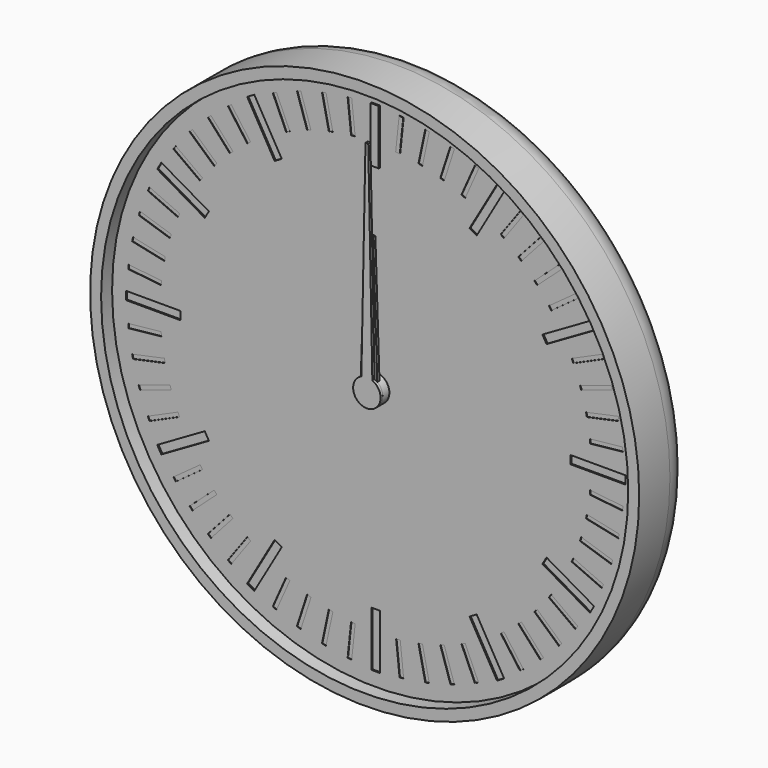
from build123d import *

# Parameters (mm, degrees)
F0_R      = 100
F1_DEPTH  = 24
F2_R      = 10
F3_T      = -4
F4_R      = 5
F4_R_2    = 3
F5_DEPTH  = 2
F6_DEPTH  = 19
F7_DEPTH  = 8
F9_DEPTH  = 4
F11_DEPTH = 4
F12_R     = 5
F12_R_2   = 3
F13_DEPTH = 2
F14_R     = 3
F15_DEPTH = 4
F17_DEPTH = 4
F18_R     = 3
F19_DEPTH = 2
F20_R     = 98
F20_R_2   = 5
F21_DEPTH = 1
F23_R     = 5
F23_R_2   = 3
F24_DEPTH = 2
F25_W     = 3
F25_H     = 20
F25_W_2   = 20
F25_H_2   = 3
F26_DEPTH = 0.5
F27_W     = 1.5
F27_H     = 12
F27_W_2   = 12
F27_H_2   = 1.5
F28_DEPTH = 0.2
F29_DEPTH = 1
F30_DEPTH = 0.4
F31_R     = 5
F31_R_2   = 3
F32_DEPTH = 5
F33_R     = 3
F34_DEPTH = 1
F36_DEPTH = 1


with BuildPart() as f1:
    # F0 (on Front) → F1 (new body)
    with BuildSketch(Plane.XZ):
        Circle(F0_R)
    extrude(amount=F1_DEPTH)

    # F2
    f2_edges = [f1.edges().sort_by_distance(p)[0] for p in [
        (-100, 0, 0),
    ]]
    fillet(f2_edges, radius=F2_R)

    # F3
    f3_openings = [f1.faces().sort_by_distance(p)[0] for p in [
        (0, -24, 0),
    ]]
    offset(amount=F3_T, openings=f3_openings)

    # F4 (on face) → F5 (join)
    with BuildSketch(Plane.XZ.offset(4)):
        Circle(F4_R)
        Circle(F4_R_2, mode=Mode.SUBTRACT)
        with Locations((40, 0)):
            Circle(F4_R)
        with Locations((40, 0)):
            Circle(F4_R_2, mode=Mode.SUBTRACT)
    extrude(amount=F5_DEPTH)


with BuildPart() as f6:
    # F6 (new): a face of the model
    f6_faces = [f1.part.faces().sort_by_distance(p)[0] for p in [
        (0, -4, 0),
    ]]
    extrude(f6_faces, amount=F6_DEPTH)

    # F8 (on face) → F9 (join)
    with BuildSketch(Plane.XZ.offset(6)):
        with BuildLine():
            ThreePointArc((9.2729637667, -1.3794085621), (9.3494561423, -0.6915886375), (9.375, 0))
            ThreePointArc((9.375, 0), (9.3494561423, 0.6915886375), (9.2729637667, 1.3794085621))
            ThreePointArc((9.2729637667, 1.3794085621), (8.9161548403, 2.8970343223), (8.3127812852, 4.3345463782))
            ThreePointArc((8.3127812852, 4.3345463782), (7.5845343223, 5.5104867402), (6.6911892658, 6.566476316))
            ThreePointArc((6.6911892658, 6.566476316), (5.5104867402, 7.5845343223), (4.1773988938, 8.3928519278))
            ThreePointArc((4.1773988938, 8.3928519278), (2.8970343223, 8.9161548403), (1.5536078905, 9.2453733036))
            ThreePointArc((1.5536078905, 9.2453733036), (0, 9.375), (-1.5536078905, 9.2453733036))
            ThreePointArc((-1.5536078905, 9.2453733036), (-2.8970343223, 8.9161548403), (-4.1773988938, 8.3928519278))
            ThreePointArc((-4.1773988938, 8.3928519278), (-5.5104867402, 7.5845343223), (-6.6911892658, 6.566476316))
            ThreePointArc((-6.6911892658, 6.566476316), (-7.5845343223, 5.5104867402), (-8.3127812852, 4.3345463782))
            ThreePointArc((-8.3127812852, 4.3345463782), (-8.9161548403, 2.8970343223), (-9.2729637667, 1.3794085621))
            ThreePointArc((-9.2729637667, 1.3794085621), (-9.375, 0), (-9.2729637667, -1.3794085621))
            ThreePointArc((-9.2729637667, -1.3794085621), (-8.9161548403, -2.8970343223), (-8.3127812852, -4.3345463782))
            ThreePointArc((-8.3127812852, -4.3345463782), (-7.5845343223, -5.5104867402), (-6.6911892658, -6.566476316))
            ThreePointArc((-6.6911892658, -6.566476316), (-5.5104867402, -7.5845343223), (-4.1773988938, -8.3928519278))
            ThreePointArc((-4.1773988938, -8.3928519278), (-2.8970343223, -8.9161548403), (-1.5536078905, -9.2453733036))
            ThreePointArc((-1.5536078905, -9.2453733036), (0, -9.375), (1.5536078905, -9.2453733036))
            ThreePointArc((1.5536078905, -9.2453733036), (2.8970343223, -8.9161548403), (4.1773988938, -8.3928519278))
            ThreePointArc((4.1773988938, -8.3928519278), (5.5104867402, -7.5845343223), (6.6911892658, -6.566476316))
            ThreePointArc((6.6911892658, -6.566476316), (7.5845343223, -5.5104867402), (8.3127812852, -4.3345463782))
            ThreePointArc((8.3127812852, -4.3345463782), (8.9161548403, -2.8970343223), (9.2729637667, -1.3794085621))
        make_face()
        with BuildLine():
            ThreePointArc((8.3127812852, 4.3345463782), (8.9161548403, 2.8970343223), (9.2729637667, 1.3794085621))
            Line((9.2729637667, 1.3794085621), (11.1823199426, 2.3946312492))
            Line((11.1823199426, 2.3946312492), (10.8182678729, 3.515068311))
            Line((10.8182678729, 3.515068311), (10.4542158031, 4.6355053728))
            Line((10.4542158031, 4.6355053728), (8.3127812852, 4.3345463782))
        make_face()
        with BuildLine():
            Line((11.1823199426, -2.3946312492), (9.2729637667, -1.3794085621))
            ThreePointArc((9.2729637667, -1.3794085621), (8.9161548403, -2.8970343223), (8.3127812852, -4.3345463782))
            Line((8.3127812852, -4.3345463782), (10.4542158031, -4.6355053728))
            Line((10.4542158031, -4.6355053728), (10.8182678729, -3.515068311))
            Line((10.8182678729, -3.515068311), (11.1823199426, -2.3946312492))
        make_face()
        with BuildLine():
            ThreePointArc((4.1773988938, 8.3928519278), (5.5104867402, 7.5845343223), (6.6911892658, 6.566476316))
            Line((6.6911892658, 6.566476316), (7.6391579371, 8.5101001246))
            Line((7.6391579371, 8.5101001246), (6.6860572448, 9.202568311))
            Line((6.6860572448, 9.202568311), (5.7329565525, 9.8950364974))
            Line((5.7329565525, 9.8950364974), (4.1773988938, 8.3928519278))
        make_face()
        with BuildLine():
            Line((7.6391579371, -8.5101001246), (6.6911892658, -6.566476316))
            ThreePointArc((6.6911892658, -6.566476316), (5.5104867402, -7.5845343223), (4.1773988938, -8.3928519278))
            Line((4.1773988938, -8.3928519278), (5.7329565525, -9.8950364974))
            Line((5.7329565525, -9.8950364974), (6.6860572448, -9.202568311))
            Line((6.6860572448, -9.202568311), (7.6391579371, -8.5101001246))
        make_face()
        with BuildLine():
            ThreePointArc((-1.5536078905, 9.2453733036), (0, 9.375), (1.5536078905, 9.2453733036))
            Line((1.5536078905, 9.2453733036), (1.1780972451, 11.375))
            Line((1.1780972451, 11.375), (0, 11.375))
            Line((0, 11.375), (-1.1780972451, 11.375))
            Line((-1.1780972451, 11.375), (-1.5536078905, 9.2453733036))
        make_face()
        with BuildLine():
            Line((1.1780972451, -11.375), (1.5536078905, -9.2453733036))
            ThreePointArc((1.5536078905, -9.2453733036), (0, -9.375), (-1.5536078905, -9.2453733036))
            Line((-1.5536078905, -9.2453733036), (-1.1780972451, -11.375))
            Line((-1.1780972451, -11.375), (0, -11.375))
            Line((0, -11.375), (1.1780972451, -11.375))
        make_face()
        with BuildLine():
            ThreePointArc((-6.6911892658, 6.566476316), (-5.5104867402, 7.5845343223), (-4.1773988938, 8.3928519278))
            Line((-4.1773988938, 8.3928519278), (-5.7329565525, 9.8950364974))
            Line((-5.7329565525, 9.8950364974), (-6.6860572448, 9.202568311))
            Line((-6.6860572448, 9.202568311), (-7.6391579371, 8.5101001246))
            Line((-7.6391579371, 8.5101001246), (-6.6911892658, 6.566476316))
        make_face()
        with BuildLine():
            Line((-5.7329565525, -9.8950364974), (-4.1773988938, -8.3928519278))
            ThreePointArc((-4.1773988938, -8.3928519278), (-5.5104867402, -7.5845343223), (-6.6911892658, -6.566476316))
            Line((-6.6911892658, -6.566476316), (-7.6391579371, -8.5101001246))
            Line((-7.6391579371, -8.5101001246), (-6.6860572448, -9.202568311))
            Line((-6.6860572448, -9.202568311), (-5.7329565525, -9.8950364974))
        make_face()
        with BuildLine():
            ThreePointArc((-9.2729637667, 1.3794085621), (-8.9161548403, 2.8970343223), (-8.3127812852, 4.3345463782))
            Line((-8.3127812852, 4.3345463782), (-10.4542158031, 4.6355053728))
            Line((-10.4542158031, 4.6355053728), (-10.8182678729, 3.515068311))
            Line((-10.8182678729, 3.515068311), (-11.1823199426, 2.3946312492))
            Line((-11.1823199426, 2.3946312492), (-9.2729637667, 1.3794085621))
        make_face()
        with BuildLine():
            Line((-10.4542158031, -4.6355053728), (-8.3127812852, -4.3345463782))
            ThreePointArc((-8.3127812852, -4.3345463782), (-8.9161548403, -2.8970343223), (-9.2729637667, -1.3794085621))
            Line((-9.2729637667, -1.3794085621), (-11.1823199426, -2.3946312492))
            Line((-11.1823199426, -2.3946312492), (-10.8182678729, -3.515068311))
            Line((-10.8182678729, -3.515068311), (-10.4542158031, -4.6355053728))
        make_face()
    extrude(amount=F9_DEPTH)

    # F35 (on face) → F36 (join)
    with BuildSketch(Plane.XZ.offset(23)):
        with BuildLine():
            ThreePointArc((-2, 4.582575695), (-2.7386127875, -4.1833001327), (5, 0))
            ThreePointArc((5, 0), (4.1833001327, 2.7386127875), (2, 4.582575695))
            ThreePointArc((2, 4.582575695), (0, 5), (-2, 4.582575695))
        make_face()
        with BuildLine():
            ThreePointArc((-2, 4.582575695), (0, 5), (2, 4.582575695))
            Line((2, 4.582575695), (0.5, 80))
            Line((0.5, 80), (0, 80))
            Line((0, 80), (-0.5, 80))
            Line((-0.5, 80), (-2, 4.582575695))
        make_face()
    extrude(amount=-F36_DEPTH)


with BuildPart() as f7:
    # F7 (new): a face of the model
    f7_faces = [f1.part.faces().sort_by_distance(p)[0] for p in [
        (40, -4, 0),
    ]]
    extrude(f7_faces, amount=F7_DEPTH)

    # F10 (on face) → F11 (join)
    with BuildSketch(Plane.XZ.offset(6)):
        with BuildLine():
            ThreePointArc((68.0829066802, -1.5381733945), (68.1144747006, -0.7693746225), (68.125, 0))
            ThreePointArc((68.125, 0), (68.1144747006, 0.7693746225), (68.0829066802, 1.5381733945))
            ThreePointArc((68.0829066802, 1.5381733945), (67.9709283072, 2.9398630294), (67.7890320221, 4.3342039956))
            ThreePointArc((67.7890320221, 4.3342039956), (67.5104012706, 5.8475163042), (67.1494235596, 7.3433252263))
            ThreePointArc((67.1494235596, 7.3433252263), (66.7484645208, 8.6911029668), (66.280643318, 10.0171558733))
            ThreePointArc((66.280643318, 10.0171558733), (65.6934659962, 11.4394680865), (65.0293803521, 12.8275385085))
            ThreePointArc((65.0293803521, 12.8275385085), (64.3569644814, 14.0625), (63.6236643925, 15.2623099717))
            ThreePointArc((63.6236643925, 15.2623099717), (62.7536029668, 16.5314602207), (61.815433119, 17.7511268046))
            ThreePointArc((61.815433119, 17.7511268046), (60.9009482166, 18.8192983038), (59.934217974, 19.8404278876))
            ThreePointArc((59.934217974, 19.8404278876), (58.8192983038, 20.9009482166), (57.6480467764, 21.8989056799))
            ThreePointArc((57.6480467764, 21.8989056799), (56.5314602207, 22.7536029668), (55.3735505752, 23.5514238999))
            ThreePointArc((55.3735505752, 23.5514238999), (54.0625, 24.3569644814), (52.709356105, 25.0895972944))
            ThreePointArc((52.709356105, 25.0895972944), (51.4394680865, 25.6934659962), (50.1409852457, 26.2331096755))
            ThreePointArc((50.1409852457, 26.2331096755), (48.6911029668, 26.7484645208), (47.2152055856, 27.1837531139))
            ThreePointArc((47.2152055856, 27.1837531139), (45.8475163042, 27.5104012706), (44.4652101991, 27.7682826779))
            ThreePointArc((44.4652101991, 27.7682826779), (42.9398630294, 27.9709283072), (41.4057159597, 28.0898484802))
            ThreePointArc((41.4057159597, 28.0898484802), (40, 28.125), (38.5942840403, 28.0898484802))
            ThreePointArc((38.5942840403, 28.0898484802), (37.0601369706, 27.9709283072), (35.5347898009, 27.7682826779))
            ThreePointArc((35.5347898009, 27.7682826779), (34.1524836958, 27.5104012706), (32.7847944144, 27.1837531139))
            ThreePointArc((32.7847944144, 27.1837531139), (31.3088970332, 26.7484645208), (29.8590147543, 26.2331096755))
            ThreePointArc((29.8590147543, 26.2331096755), (28.5605319135, 25.6934659962), (27.290643895, 25.0895972944))
            ThreePointArc((27.290643895, 25.0895972944), (25.9375, 24.3569644814), (24.6264494248, 23.5514238999))
            ThreePointArc((24.6264494248, 23.5514238999), (23.4685397793, 22.7536029668), (22.3519532236, 21.8989056799))
            ThreePointArc((22.3519532236, 21.8989056799), (21.1807016962, 20.9009482166), (20.065782026, 19.8404278876))
            ThreePointArc((20.065782026, 19.8404278876), (19.0990517834, 18.8192983038), (18.184566881, 17.7511268046))
            ThreePointArc((18.184566881, 17.7511268046), (17.2463970332, 16.5314602207), (16.3763356075, 15.2623099717))
            ThreePointArc((16.3763356075, 15.2623099717), (15.6430355186, 14.0625), (14.9706196479, 12.8275385085))
            ThreePointArc((14.9706196479, 12.8275385085), (14.3065340038, 11.4394680865), (13.719356682, 10.0171558733))
            ThreePointArc((13.719356682, 10.0171558733), (13.2515354792, 8.6911029668), (12.8505764404, 7.3433252263))
            ThreePointArc((12.8505764404, 7.3433252263), (12.4895987294, 5.8475163042), (12.2109679779, 4.3342039956))
            ThreePointArc((12.2109679779, 4.3342039956), (12.0290716928, 2.9398630294), (11.9170933198, 1.5381733945))
            ThreePointArc((11.9170933198, 1.5381733945), (11.875, 0), (11.9170933198, -1.5381733945))
            ThreePointArc((11.9170933198, -1.5381733945), (12.0290716928, -2.9398630294), (12.2109679779, -4.3342039956))
            ThreePointArc((12.2109679779, -4.3342039956), (12.4895987294, -5.8475163042), (12.8505764404, -7.3433252263))
            ThreePointArc((12.8505764404, -7.3433252263), (13.2515354792, -8.6911029668), (13.719356682, -10.0171558733))
            ThreePointArc((13.719356682, -10.0171558733), (14.3065340038, -11.4394680865), (14.9706196479, -12.8275385085))
            ThreePointArc((14.9706196479, -12.8275385085), (15.6430355186, -14.0625), (16.3763356075, -15.2623099717))
            ThreePointArc((16.3763356075, -15.2623099717), (17.2463970332, -16.5314602207), (18.184566881, -17.7511268046))
            ThreePointArc((18.184566881, -17.7511268046), (19.0990517834, -18.8192983038), (20.065782026, -19.8404278876))
            ThreePointArc((20.065782026, -19.8404278876), (21.1807016962, -20.9009482166), (22.3519532236, -21.8989056799))
            ThreePointArc((22.3519532236, -21.8989056799), (23.4685397793, -22.7536029668), (24.6264494248, -23.5514238999))
            ThreePointArc((24.6264494248, -23.5514238999), (25.9375, -24.3569644814), (27.290643895, -25.0895972944))
            ThreePointArc((27.290643895, -25.0895972944), (28.5605319135, -25.6934659962), (29.8590147543, -26.2331096755))
            ThreePointArc((29.8590147543, -26.2331096755), (31.3088970332, -26.7484645208), (32.7847944144, -27.1837531139))
            ThreePointArc((32.7847944144, -27.1837531139), (34.1524836958, -27.5104012706), (35.5347898009, -27.7682826779))
            ThreePointArc((35.5347898009, -27.7682826779), (37.0601369706, -27.9709283072), (38.5942840403, -28.0898484802))
            ThreePointArc((38.5942840403, -28.0898484802), (40, -28.125), (41.4057159597, -28.0898484802))
            ThreePointArc((41.4057159597, -28.0898484802), (42.9398630294, -27.9709283072), (44.4652101991, -27.7682826779))
            ThreePointArc((44.4652101991, -27.7682826779), (45.8475163042, -27.5104012706), (47.2152055856, -27.1837531139))
            ThreePointArc((47.2152055856, -27.1837531139), (48.6911029668, -26.7484645208), (50.1409852457, -26.2331096755))
            ThreePointArc((50.1409852457, -26.2331096755), (51.4394680865, -25.6934659962), (52.709356105, -25.0895972944))
            ThreePointArc((52.709356105, -25.0895972944), (54.0625, -24.3569644814), (55.3735505752, -23.5514238999))
            ThreePointArc((55.3735505752, -23.5514238999), (56.5314602207, -22.7536029668), (57.6480467764, -21.8989056799))
            ThreePointArc((57.6480467764, -21.8989056799), (58.8192983038, -20.9009482166), (59.934217974, -19.8404278876))
            ThreePointArc((59.934217974, -19.8404278876), (60.9009482166, -18.8192983038), (61.815433119, -17.7511268046))
            ThreePointArc((61.815433119, -17.7511268046), (62.7536029668, -16.5314602207), (63.6236643925, -15.2623099717))
            ThreePointArc((63.6236643925, -15.2623099717), (64.3569644814, -14.0625), (65.0293803521, -12.8275385085))
            ThreePointArc((65.0293803521, -12.8275385085), (65.6934659962, -11.4394680865), (66.280643318, -10.0171558733))
            ThreePointArc((66.280643318, -10.0171558733), (66.7484645208, -8.6911029668), (67.1494235596, -7.3433252263))
            ThreePointArc((67.1494235596, -7.3433252263), (67.5104012706, -5.8475163042), (67.7890320221, -4.3342039956))
            ThreePointArc((67.7890320221, -4.3342039956), (67.9709283072, -2.9398630294), (68.0829066802, -1.5381733945))
        make_face()
        with BuildLine():
            ThreePointArc((68.0829066802, 1.5381733945), (68.1144747006, 0.7693746225), (68.125, 0))
            ThreePointArc((68.125, 0), (68.1144747006, -0.7693746225), (68.0829066802, -1.5381733945))
            Line((68.0829066802, -1.5381733945), (70.125, -1.1780972451))
            Line((70.125, -1.1780972451), (70.125, 0))
            Line((70.125, 0), (70.125, 1.1780972451))
            Line((70.125, 1.1780972451), (68.0829066802, 1.5381733945))
        make_face()
        with BuildLine():
            ThreePointArc((67.1494235596, 7.3433252263), (67.5104012706, 5.8475163042), (67.7890320221, 4.3342039956))
            Line((67.7890320221, 4.3342039956), (69.7116366623, 5.1109866922))
            Line((69.7116366623, 5.1109866922), (69.4666964721, 6.2633396859))
            Line((69.4666964721, 6.2633396859), (69.2217562819, 7.4156926796))
            Line((69.2217562819, 7.4156926796), (67.1494235596, 7.3433252263))
        make_face()
        with BuildLine():
            Line((69.7116366623, -5.1109866922), (67.7890320221, -4.3342039956))
            ThreePointArc((67.7890320221, -4.3342039956), (67.5104012706, -5.8475163042), (67.1494235596, -7.3433252263))
            Line((67.1494235596, -7.3433252263), (69.2217562819, -7.4156926796))
            Line((69.2217562819, -7.4156926796), (69.4666964721, -6.2633396859))
            Line((69.4666964721, -6.2633396859), (69.7116366623, -5.1109866922))
        make_face()
        with BuildLine():
            ThreePointArc((65.0293803521, 12.8275385085), (65.6934659962, 11.4394680865), (66.280643318, 10.0171558733))
            Line((66.280643318, 10.0171558733), (67.9997322302, 11.1766959857))
            Line((67.9997322302, 11.1766959857), (67.5205569115, 12.2529413727))
            Line((67.5205569115, 12.2529413727), (67.0413815928, 13.3291867596))
            Line((67.0413815928, 13.3291867596), (65.0293803521, 12.8275385085))
        make_face()
        with BuildLine():
            Line((67.9997322302, -11.1766959857), (66.280643318, -10.0171558733))
            ThreePointArc((66.280643318, -10.0171558733), (65.6934659962, -11.4394680865), (65.0293803521, -12.8275385085))
            Line((65.0293803521, -12.8275385085), (67.0413815928, -13.3291867596))
            Line((67.0413815928, -13.3291867596), (67.5205569115, -12.2529413727))
            Line((67.5205569115, -12.2529413727), (67.9997322302, -11.1766959857))
        make_face()
        with BuildLine():
            ThreePointArc((61.815433119, 17.7511268046), (62.7536029668, 16.5314602207), (63.6236643925, 15.2623099717))
            Line((63.6236643925, 15.2623099717), (65.064105142, 16.753930033))
            Line((65.064105142, 16.753930033), (64.3716369555, 17.7070307253))
            Line((64.3716369555, 17.7070307253), (63.6791687691, 18.6601314176))
            Line((63.6791687691, 18.6601314176), (61.815433119, 17.7511268046))
        make_face()
        with BuildLine():
            Line((65.064105142, -16.753930033), (63.6236643925, -15.2623099717))
            ThreePointArc((63.6236643925, -15.2623099717), (62.7536029668, -16.5314602207), (61.815433119, -17.7511268046))
            Line((61.815433119, -17.7511268046), (63.6791687691, -18.6601314176))
            Line((63.6791687691, -18.6601314176), (64.3716369555, -17.7070307253))
            Line((64.3716369555, -17.7070307253), (65.064105142, -16.753930033))
        make_face()
        with BuildLine():
            ThreePointArc((57.6480467764, 21.8989056799), (58.8192983038, 20.9009482166), (59.934217974, 19.8404278876))
            Line((59.934217974, 19.8404278876), (61.0330563882, 21.5989369435))
            Line((61.0330563882, 21.5989369435), (60.1575595166, 22.3872378675))
            Line((60.1575595166, 22.3872378675), (59.282062645, 23.1755387915))
            Line((59.282062645, 23.1755387915), (57.6480467764, 21.8989056799))
        make_face()
        with BuildLine():
            Line((61.0330563882, -21.5989369435), (59.934217974, -19.8404278876))
            ThreePointArc((59.934217974, -19.8404278876), (58.8192983038, -20.9009482166), (57.6480467764, -21.8989056799))
            Line((57.6480467764, -21.8989056799), (59.282062645, -23.1755387915))
            Line((59.282062645, -23.1755387915), (60.1575595166, -22.3872378675))
            Line((60.1575595166, -22.3872378675), (61.0330563882, -21.5989369435))
        make_face()
        with BuildLine():
            ThreePointArc((52.709356105, 25.0895972944), (54.0625, 24.3569644814), (55.3735505752, 23.5514238999))
            Line((55.3735505752, 23.5514238999), (56.0827621424, 25.4999666665))
            Line((56.0827621424, 25.4999666665), (55.0625, 26.089015289))
            Line((55.0625, 26.089015289), (54.0422378576, 26.6780639116))
            Line((54.0422378576, 26.6780639116), (52.709356105, 25.0895972944))
        make_face()
        with BuildLine():
            Line((56.0827621424, -25.4999666665), (55.3735505752, -23.5514238999))
            ThreePointArc((55.3735505752, -23.5514238999), (54.0625, -24.3569644814), (52.709356105, -25.0895972944))
            Line((52.709356105, -25.0895972944), (54.0422378576, -26.6780639116))
            Line((54.0422378576, -26.6780639116), (55.0625, -26.089015289))
            Line((55.0625, -26.089015289), (56.0827621424, -25.4999666665))
        make_face()
        with BuildLine():
            ThreePointArc((47.2152055856, 27.1837531139), (48.6911029668, 26.7484645208), (50.1409852457, 26.2331096755))
            Line((50.1409852457, 26.2331096755), (50.4295740173, 28.2865254836))
            Line((50.4295740173, 28.2865254836), (49.3091369555, 28.6505775534))
            Line((49.3091369555, 28.6505775534), (48.1886998938, 29.0146296232))
            Line((48.1886998938, 29.0146296232), (47.2152055856, 27.1837531139))
        make_face()
        with BuildLine():
            Line((50.4295740173, -28.2865254836), (50.1409852457, -26.2331096755))
            ThreePointArc((50.1409852457, -26.2331096755), (48.6911029668, -26.7484645208), (47.2152055856, -27.1837531139))
            Line((47.2152055856, -27.1837531139), (48.1886998938, -29.0146296232))
            Line((48.1886998938, -29.0146296232), (49.3091369555, -28.6505775534))
            Line((49.3091369555, -28.6505775534), (50.4295740173, -28.2865254836))
        make_face()
        with BuildLine():
            ThreePointArc((41.4057159597, 28.0898484802), (42.9398630294, 27.9709283072), (44.4652101991, 27.7682826779))
            Line((44.4652101991, 27.7682826779), (44.3205634611, 29.8368274034))
            Line((44.3205634611, 29.8368274034), (43.1489199559, 29.959972098))
            Line((43.1489199559, 29.959972098), (41.9772764508, 30.0831167926))
            Line((41.9772764508, 30.0831167926), (41.4057159597, 28.0898484802))
        make_face()
        with BuildLine():
            Line((44.3205634611, -29.8368274034), (44.4652101991, -27.7682826779))
            ThreePointArc((44.4652101991, -27.7682826779), (42.9398630294, -27.9709283072), (41.4057159597, -28.0898484802))
            Line((41.4057159597, -28.0898484802), (41.9772764508, -30.0831167926))
            Line((41.9772764508, -30.0831167926), (43.1489199559, -29.959972098))
            Line((43.1489199559, -29.959972098), (44.3205634611, -29.8368274034))
        make_face()
        with BuildLine():
            ThreePointArc((35.5347898009, 27.7682826779), (37.0601369706, 27.9709283072), (38.5942840403, 28.0898484802))
            Line((38.5942840403, 28.0898484802), (38.0227235492, 30.0831167926))
            Line((38.0227235492, 30.0831167926), (36.8510800441, 29.959972098))
            Line((36.8510800441, 29.959972098), (35.6794365389, 29.8368274034))
            Line((35.6794365389, 29.8368274034), (35.5347898009, 27.7682826779))
        make_face()
        with BuildLine():
            Line((38.0227235492, -30.0831167926), (38.5942840403, -28.0898484802))
            ThreePointArc((38.5942840403, -28.0898484802), (37.0601369706, -27.9709283072), (35.5347898009, -27.7682826779))
            Line((35.5347898009, -27.7682826779), (35.6794365389, -29.8368274034))
            Line((35.6794365389, -29.8368274034), (36.8510800441, -29.959972098))
            Line((36.8510800441, -29.959972098), (38.0227235492, -30.0831167926))
        make_face()
        with BuildLine():
            ThreePointArc((29.8590147543, 26.2331096755), (31.3088970332, 26.7484645208), (32.7847944144, 27.1837531139))
            Line((32.7847944144, 27.1837531139), (31.8113001062, 29.0146296232))
            Line((31.8113001062, 29.0146296232), (30.6908630445, 28.6505775534))
            Line((30.6908630445, 28.6505775534), (29.5704259827, 28.2865254836))
            Line((29.5704259827, 28.2865254836), (29.8590147543, 26.2331096755))
        make_face()
        with BuildLine():
            Line((31.8113001062, -29.0146296232), (32.7847944144, -27.1837531139))
            ThreePointArc((32.7847944144, -27.1837531139), (31.3088970332, -26.7484645208), (29.8590147543, -26.2331096755))
            Line((29.8590147543, -26.2331096755), (29.5704259827, -28.2865254836))
            Line((29.5704259827, -28.2865254836), (30.6908630445, -28.6505775534))
            Line((30.6908630445, -28.6505775534), (31.8113001062, -29.0146296232))
        make_face()
        with BuildLine():
            ThreePointArc((24.6264494248, 23.5514238999), (25.9375, 24.3569644814), (27.290643895, 25.0895972944))
            Line((27.290643895, 25.0895972944), (25.9577621424, 26.6780639116))
            Line((25.9577621424, 26.6780639116), (24.9375, 26.089015289))
            Line((24.9375, 26.089015289), (23.9172378576, 25.4999666665))
            Line((23.9172378576, 25.4999666665), (24.6264494248, 23.5514238999))
        make_face()
        with BuildLine():
            Line((25.9577621424, -26.6780639116), (27.290643895, -25.0895972944))
            ThreePointArc((27.290643895, -25.0895972944), (25.9375, -24.3569644814), (24.6264494248, -23.5514238999))
            Line((24.6264494248, -23.5514238999), (23.9172378576, -25.4999666665))
            Line((23.9172378576, -25.4999666665), (24.9375, -26.089015289))
            Line((24.9375, -26.089015289), (25.9577621424, -26.6780639116))
        make_face()
        with BuildLine():
            ThreePointArc((20.065782026, 19.8404278876), (21.1807016962, 20.9009482166), (22.3519532236, 21.8989056799))
            Line((22.3519532236, 21.8989056799), (20.717937355, 23.1755387915))
            Line((20.717937355, 23.1755387915), (19.8424404834, 22.3872378675))
            Line((19.8424404834, 22.3872378675), (18.9669436118, 21.5989369435))
            Line((18.9669436118, 21.5989369435), (20.065782026, 19.8404278876))
        make_face()
        with BuildLine():
            Line((20.717937355, -23.1755387915), (22.3519532236, -21.8989056799))
            ThreePointArc((22.3519532236, -21.8989056799), (21.1807016962, -20.9009482166), (20.065782026, -19.8404278876))
            Line((20.065782026, -19.8404278876), (18.9669436118, -21.5989369435))
            Line((18.9669436118, -21.5989369435), (19.8424404834, -22.3872378675))
            Line((19.8424404834, -22.3872378675), (20.717937355, -23.1755387915))
        make_face()
        with BuildLine():
            ThreePointArc((16.3763356075, 15.2623099717), (17.2463970332, 16.5314602207), (18.184566881, 17.7511268046))
            Line((18.184566881, 17.7511268046), (16.3208312309, 18.6601314176))
            Line((16.3208312309, 18.6601314176), (15.6283630445, 17.7070307253))
            Line((15.6283630445, 17.7070307253), (14.935894858, 16.753930033))
            Line((14.935894858, 16.753930033), (16.3763356075, 15.2623099717))
        make_face()
        with BuildLine():
            Line((16.3208312309, -18.6601314176), (18.184566881, -17.7511268046))
            ThreePointArc((18.184566881, -17.7511268046), (17.2463970332, -16.5314602207), (16.3763356075, -15.2623099717))
            Line((16.3763356075, -15.2623099717), (14.935894858, -16.753930033))
            Line((14.935894858, -16.753930033), (15.6283630445, -17.7070307253))
            Line((15.6283630445, -17.7070307253), (16.3208312309, -18.6601314176))
        make_face()
        with BuildLine():
            ThreePointArc((13.719356682, 10.0171558733), (14.3065340038, 11.4394680865), (14.9706196479, 12.8275385085))
            Line((14.9706196479, 12.8275385085), (12.9586184072, 13.3291867596))
            Line((12.9586184072, 13.3291867596), (12.4794430885, 12.2529413727))
            Line((12.4794430885, 12.2529413727), (12.0002677698, 11.1766959857))
            Line((12.0002677698, 11.1766959857), (13.719356682, 10.0171558733))
        make_face()
        with BuildLine():
            Line((12.9586184072, -13.3291867596), (14.9706196479, -12.8275385085))
            ThreePointArc((14.9706196479, -12.8275385085), (14.3065340038, -11.4394680865), (13.719356682, -10.0171558733))
            Line((13.719356682, -10.0171558733), (12.0002677698, -11.1766959857))
            Line((12.0002677698, -11.1766959857), (12.4794430885, -12.2529413727))
            Line((12.4794430885, -12.2529413727), (12.9586184072, -13.3291867596))
        make_face()
        with BuildLine():
            ThreePointArc((12.2109679779, 4.3342039956), (12.4895987294, 5.8475163042), (12.8505764404, 7.3433252263))
            Line((12.8505764404, 7.3433252263), (10.7782437181, 7.4156926796))
            Line((10.7782437181, 7.4156926796), (10.5333035279, 6.2633396859))
            Line((10.5333035279, 6.2633396859), (10.2883633377, 5.1109866922))
            Line((10.2883633377, 5.1109866922), (12.2109679779, 4.3342039956))
        make_face()
        with BuildLine():
            Line((10.7782437181, -7.4156926796), (12.8505764404, -7.3433252263))
            ThreePointArc((12.8505764404, -7.3433252263), (12.4895987294, -5.8475163042), (12.2109679779, -4.3342039956))
            Line((12.2109679779, -4.3342039956), (10.2883633377, -5.1109866922))
            Line((10.2883633377, -5.1109866922), (10.5333035279, -6.2633396859))
            Line((10.5333035279, -6.2633396859), (10.7782437181, -7.4156926796))
        make_face()
        with BuildLine():
            ThreePointArc((11.9170933198, -1.5381733945), (11.875, 0), (11.9170933198, 1.5381733945))
            Line((11.9170933198, 1.5381733945), (9.875, 1.1780972451))
            Line((9.875, 1.1780972451), (9.875, 0))
            Line((9.875, 0), (9.875, -1.1780972451))
            Line((9.875, -1.1780972451), (11.9170933198, -1.5381733945))
        make_face()
    extrude(amount=F11_DEPTH)

    # F16 (on face) → F17 (join)
    with BuildSketch(Plane.XZ.offset(12)):
        with BuildLine():
            ThreePointArc((47.4288750323, -1.0304444454), (47.4821976298, -0.5164480894), (47.5, 0))
            ThreePointArc((47.5, 0), (47.4821976298, 0.5164480894), (47.4288750323, 1.0304444454))
            ThreePointArc((47.4288750323, 1.0304444454), (47.1329238722, 2.3176274578), (46.6157661985, 3.532936117))
            ThreePointArc((46.6157661985, 3.532936117), (46.0676274578, 4.4083893922), (45.4044061018, 5.2002302532))
            ThreePointArc((45.4044061018, 5.2002302532), (44.4083893922, 6.0676274578), (43.2756595386, 6.7468551628))
            ThreePointArc((43.2756595386, 6.7468551628), (42.3176274578, 7.1329238722), (41.3156377295, 7.3837048536))
            ThreePointArc((41.3156377295, 7.3837048536), (40, 7.5), (38.6843622705, 7.3837048536))
            ThreePointArc((38.6843622705, 7.3837048536), (37.6823725422, 7.1329238722), (36.7243404614, 6.7468551628))
            ThreePointArc((36.7243404614, 6.7468551628), (35.5916106078, 6.0676274578), (34.5955938982, 5.2002302532))
            ThreePointArc((34.5955938982, 5.2002302532), (33.9323725422, 4.4083893922), (33.3842338015, 3.532936117))
            ThreePointArc((33.3842338015, 3.532936117), (32.8670761278, 2.3176274578), (32.5711249677, 1.0304444454))
            ThreePointArc((32.5711249677, 1.0304444454), (32.5, 0), (32.5711249677, -1.0304444454))
            ThreePointArc((32.5711249677, -1.0304444454), (32.8670761278, -2.3176274578), (33.3842338015, -3.532936117))
            ThreePointArc((33.3842338015, -3.532936117), (33.9323725422, -4.4083893922), (34.5955938982, -5.2002302532))
            ThreePointArc((34.5955938982, -5.2002302532), (35.5916106078, -6.0676274578), (36.7243404614, -6.7468551628))
            ThreePointArc((36.7243404614, -6.7468551628), (37.6823725422, -7.1329238722), (38.6843622705, -7.3837048536))
            ThreePointArc((38.6843622705, -7.3837048536), (40, -7.5), (41.3156377295, -7.3837048536))
            ThreePointArc((41.3156377295, -7.3837048536), (42.3176274578, -7.1329238722), (43.2756595386, -6.7468551628))
            ThreePointArc((43.2756595386, -6.7468551628), (44.4083893922, -6.0676274578), (45.4044061018, -5.2002302532))
            ThreePointArc((45.4044061018, -5.2002302532), (46.0676274578, -4.4083893922), (46.6157661985, -3.532936117))
            ThreePointArc((46.6157661985, -3.532936117), (47.1329238722, -2.3176274578), (47.4288750323, -1.0304444454))
        make_face()
        with BuildLine():
            ThreePointArc((46.6157661985, 3.532936117), (47.1329238722, 2.3176274578), (47.4288750323, 1.0304444454))
            Line((47.4288750323, 1.0304444454), (49.3262785606, 2.0393117971))
            Line((49.3262785606, 2.0393117971), (48.743795249, 3.832011096))
            Line((48.743795249, 3.832011096), (46.6157661985, 3.532936117))
        make_face()
        with BuildLine():
            Line((49.3262785606, -2.0393117971), (47.4288750323, -1.0304444454))
            ThreePointArc((47.4288750323, -1.0304444454), (47.1329238722, -2.3176274578), (46.6157661985, -3.532936117))
            Line((46.6157661985, -3.532936117), (48.743795249, -3.832011096))
            Line((48.743795249, -3.832011096), (49.3262785606, -2.0393117971))
        make_face()
        with BuildLine():
            ThreePointArc((43.2756595386, 6.7468551628), (44.4083893922, 6.0676274578), (45.4044061018, 5.2002302532))
            Line((45.4044061018, 5.2002302532), (46.3464404506, 7.1316868974))
            Line((46.3464404506, 7.1316868974), (44.8214793429, 8.2396359957))
            Line((44.8214793429, 8.2396359957), (43.2756595386, 6.7468551628))
        make_face()
        with BuildLine():
            Line((46.3464404506, -7.1316868974), (45.4044061018, -5.2002302532))
            ThreePointArc((45.4044061018, -5.2002302532), (44.4083893922, -6.0676274578), (43.2756595386, -6.7468551628))
            Line((43.2756595386, -6.7468551628), (44.8214793429, -8.2396359957))
            Line((44.8214793429, -8.2396359957), (46.3464404506, -7.1316868974))
        make_face()
        with BuildLine():
            ThreePointArc((38.6843622705, 7.3837048536), (40, 7.5), (41.3156377295, 7.3837048536))
            Line((41.3156377295, 7.3837048536), (40.9424777961, 9.5))
            Line((40.9424777961, 9.5), (39.0575222039, 9.5))
            Line((39.0575222039, 9.5), (38.6843622705, 7.3837048536))
        make_face()
        with BuildLine():
            Line((40.9424777961, -9.5), (41.3156377295, -7.3837048536))
            ThreePointArc((41.3156377295, -7.3837048536), (40, -7.5), (38.6843622705, -7.3837048536))
            Line((38.6843622705, -7.3837048536), (39.0575222039, -9.5))
            Line((39.0575222039, -9.5), (40.9424777961, -9.5))
        make_face()
        with BuildLine():
            ThreePointArc((34.5955938982, 5.2002302532), (35.5916106078, 6.0676274578), (36.7243404614, 6.7468551628))
            Line((36.7243404614, 6.7468551628), (35.1785206571, 8.2396359957))
            Line((35.1785206571, 8.2396359957), (33.6535595494, 7.1316868974))
            Line((33.6535595494, 7.1316868974), (34.5955938982, 5.2002302532))
        make_face()
        with BuildLine():
            Line((35.1785206571, -8.2396359957), (36.7243404614, -6.7468551628))
            ThreePointArc((36.7243404614, -6.7468551628), (35.5916106078, -6.0676274578), (34.5955938982, -5.2002302532))
            Line((34.5955938982, -5.2002302532), (33.6535595494, -7.1316868974))
            Line((33.6535595494, -7.1316868974), (35.1785206571, -8.2396359957))
        make_face()
        with BuildLine():
            ThreePointArc((32.5711249677, 1.0304444454), (32.8670761278, 2.3176274578), (33.3842338015, 3.532936117))
            Line((33.3842338015, 3.532936117), (31.256204751, 3.832011096))
            Line((31.256204751, 3.832011096), (30.6737214394, 2.0393117971))
            Line((30.6737214394, 2.0393117971), (32.5711249677, 1.0304444454))
        make_face()
        with BuildLine():
            Line((31.256204751, -3.832011096), (33.3842338015, -3.532936117))
            ThreePointArc((33.3842338015, -3.532936117), (32.8670761278, -2.3176274578), (32.5711249677, -1.0304444454))
            Line((32.5711249677, -1.0304444454), (30.6737214394, -2.0393117971))
            Line((30.6737214394, -2.0393117971), (31.256204751, -3.832011096))
        make_face()
    extrude(amount=F17_DEPTH)

    # F18 (on face) → F19 (join)
    with BuildSketch(Plane.XZ.offset(16)):
        with Locations((40, 0)):
            Circle(F18_R)
    extrude(amount=F19_DEPTH)


with BuildPart() as f13:
    # F12 (on face) → F13 (new body)
    with BuildSketch(Plane.XZ.offset(10)):
        Circle(F12_R)
        Circle(F12_R_2, mode=Mode.SUBTRACT)
    extrude(amount=F13_DEPTH)

    # F14 (on face) → F15 (join)
    with BuildSketch(Plane.XZ.offset(12)):
        with BuildLine():
            ThreePointArc((29.9718156995, -1.3001014101), (29.9929530972, -0.6502034357), (30, 0))
            ThreePointArc((30, 0), (29.9929530972, 0.6502034357), (29.9718156995, 1.3001014101))
            ThreePointArc((29.9718156995, 1.3001014101), (29.907520012, 2.3537728718), (29.8061935814, 3.4045299509))
            ThreePointArc((29.8061935814, 3.4045299509), (29.6306502179, 4.6930339512), (29.3994322443, 5.9727199596))
            ThreePointArc((29.3994322443, 5.9727199596), (29.1710976119, 7.0033609157), (28.9066440563, 8.0253304855))
            ThreePointArc((28.9066440563, 8.0253304855), (28.5316954889, 9.2705098312), (28.1031371961, 10.4982703213))
            ThreePointArc((28.1031371961, 10.4982703213), (27.7163859753, 11.480502971), (27.2953170189, 12.448520749))
            ThreePointArc((27.2953170189, 12.448520749), (26.7301957257, 13.6197149922), (26.1148496411, 14.765318426))
            ThreePointArc((26.1148496411, 14.765318426), (25.5792049306, 15.6749569415), (25.0118886885, 16.5651871174))
            ThreePointArc((25.0118886885, 16.5651871174), (24.2705098312, 17.6335575688), (23.4835278178, 18.6687953878))
            ThreePointArc((23.4835278178, 18.6687953878), (22.812178968, 19.4834414499), (22.1125846489, 20.2739636023))
            ThreePointArc((22.1125846489, 20.2739636023), (21.2132034356, 21.2132034356), (20.2739636023, 22.1125846489))
            ThreePointArc((20.2739636023, 22.1125846489), (19.4834414499, 22.812178968), (18.6687953878, 23.4835278178))
            ThreePointArc((18.6687953878, 23.4835278178), (17.6335575688, 24.2705098312), (16.5651871174, 25.0118886885))
            ThreePointArc((16.5651871174, 25.0118886885), (15.6749569415, 25.5792049306), (14.765318426, 26.1148496411))
            ThreePointArc((14.765318426, 26.1148496411), (13.6197149922, 26.7301957257), (12.448520749, 27.2953170189))
            ThreePointArc((12.448520749, 27.2953170189), (11.480502971, 27.7163859753), (10.4982703213, 28.1031371961))
            ThreePointArc((10.4982703213, 28.1031371961), (9.2705098312, 28.5316954889), (8.0253304855, 28.9066440563))
            ThreePointArc((8.0253304855, 28.9066440563), (7.0033609157, 29.1710976119), (5.9727199596, 29.3994322443))
            ThreePointArc((5.9727199596, 29.3994322443), (4.6930339512, 29.6306502179), (3.4045299509, 29.8061935814))
            ThreePointArc((3.4045299509, 29.8061935814), (2.3537728718, 29.907520012), (1.3001014101, 29.9718156995))
            ThreePointArc((1.3001014101, 29.9718156995), (0, 30), (-1.3001014101, 29.9718156995))
            ThreePointArc((-1.3001014101, 29.9718156995), (-2.3537728718, 29.907520012), (-3.4045299509, 29.8061935814))
            ThreePointArc((-3.4045299509, 29.8061935814), (-4.6930339512, 29.6306502179), (-5.9727199596, 29.3994322443))
            ThreePointArc((-5.9727199596, 29.3994322443), (-7.0033609157, 29.1710976119), (-8.0253304855, 28.9066440563))
            ThreePointArc((-8.0253304855, 28.9066440563), (-9.2705098312, 28.5316954889), (-10.4982703213, 28.1031371961))
            ThreePointArc((-10.4982703213, 28.1031371961), (-11.480502971, 27.7163859753), (-12.448520749, 27.2953170189))
            ThreePointArc((-12.448520749, 27.2953170189), (-13.6197149922, 26.7301957257), (-14.765318426, 26.1148496411))
            ThreePointArc((-14.765318426, 26.1148496411), (-15.6749569415, 25.5792049306), (-16.5651871174, 25.0118886885))
            ThreePointArc((-16.5651871174, 25.0118886885), (-17.6335575688, 24.2705098312), (-18.6687953878, 23.4835278178))
            ThreePointArc((-18.6687953878, 23.4835278178), (-19.4834414499, 22.812178968), (-20.2739636023, 22.1125846489))
            ThreePointArc((-20.2739636023, 22.1125846489), (-21.2132034356, 21.2132034356), (-22.1125846489, 20.2739636023))
            ThreePointArc((-22.1125846489, 20.2739636023), (-22.812178968, 19.4834414499), (-23.4835278178, 18.6687953878))
            ThreePointArc((-23.4835278178, 18.6687953878), (-24.2705098312, 17.6335575688), (-25.0118886885, 16.5651871174))
            ThreePointArc((-25.0118886885, 16.5651871174), (-25.5792049306, 15.6749569415), (-26.1148496411, 14.765318426))
            ThreePointArc((-26.1148496411, 14.765318426), (-26.7301957257, 13.6197149922), (-27.2953170189, 12.448520749))
            ThreePointArc((-27.2953170189, 12.448520749), (-27.7163859753, 11.480502971), (-28.1031371961, 10.4982703213))
            ThreePointArc((-28.1031371961, 10.4982703213), (-28.5316954889, 9.2705098312), (-28.9066440563, 8.0253304855))
            ThreePointArc((-28.9066440563, 8.0253304855), (-29.1710976119, 7.0033609157), (-29.3994322443, 5.9727199596))
            ThreePointArc((-29.3994322443, 5.9727199596), (-29.6306502179, 4.6930339512), (-29.8061935814, 3.4045299509))
            ThreePointArc((-29.8061935814, 3.4045299509), (-29.907520012, 2.3537728718), (-29.9718156995, 1.3001014101))
            ThreePointArc((-29.9718156995, 1.3001014101), (-30, 0), (-29.9718156995, -1.3001014101))
            ThreePointArc((-29.9718156995, -1.3001014101), (-29.907520012, -2.3537728718), (-29.8061935814, -3.4045299509))
            ThreePointArc((-29.8061935814, -3.4045299509), (-29.6306502179, -4.6930339512), (-29.3994322443, -5.9727199596))
            ThreePointArc((-29.3994322443, -5.9727199596), (-29.1710976119, -7.0033609157), (-28.9066440563, -8.0253304855))
            ThreePointArc((-28.9066440563, -8.0253304855), (-28.5316954889, -9.2705098312), (-28.1031371961, -10.4982703213))
            ThreePointArc((-28.1031371961, -10.4982703213), (-27.7163859753, -11.480502971), (-27.2953170189, -12.448520749))
            ThreePointArc((-27.2953170189, -12.448520749), (-26.7301957257, -13.6197149922), (-26.1148496411, -14.765318426))
            ThreePointArc((-26.1148496411, -14.765318426), (-25.5792049306, -15.6749569415), (-25.0118886885, -16.5651871174))
            ThreePointArc((-25.0118886885, -16.5651871174), (-24.2705098312, -17.6335575688), (-23.4835278178, -18.6687953878))
            ThreePointArc((-23.4835278178, -18.6687953878), (-22.812178968, -19.4834414499), (-22.1125846489, -20.2739636023))
            ThreePointArc((-22.1125846489, -20.2739636023), (-21.2132034356, -21.2132034356), (-20.2739636023, -22.1125846489))
            ThreePointArc((-20.2739636023, -22.1125846489), (-19.4834414499, -22.812178968), (-18.6687953878, -23.4835278178))
            ThreePointArc((-18.6687953878, -23.4835278178), (-17.6335575688, -24.2705098312), (-16.5651871174, -25.0118886885))
            ThreePointArc((-16.5651871174, -25.0118886885), (-15.6749569415, -25.5792049306), (-14.765318426, -26.1148496411))
            ThreePointArc((-14.765318426, -26.1148496411), (-13.6197149922, -26.7301957257), (-12.448520749, -27.2953170189))
            ThreePointArc((-12.448520749, -27.2953170189), (-11.480502971, -27.7163859753), (-10.4982703213, -28.1031371961))
            ThreePointArc((-10.4982703213, -28.1031371961), (-9.2705098312, -28.5316954889), (-8.0253304855, -28.9066440563))
            ThreePointArc((-8.0253304855, -28.9066440563), (-7.0033609157, -29.1710976119), (-5.9727199596, -29.3994322443))
            ThreePointArc((-5.9727199596, -29.3994322443), (-4.6930339512, -29.6306502179), (-3.4045299509, -29.8061935814))
            ThreePointArc((-3.4045299509, -29.8061935814), (-2.3537728718, -29.907520012), (-1.3001014101, -29.9718156995))
            ThreePointArc((-1.3001014101, -29.9718156995), (0, -30), (1.3001014101, -29.9718156995))
            ThreePointArc((1.3001014101, -29.9718156995), (2.3537728718, -29.907520012), (3.4045299509, -29.8061935814))
            ThreePointArc((3.4045299509, -29.8061935814), (4.6930339512, -29.6306502179), (5.9727199596, -29.3994322443))
            ThreePointArc((5.9727199596, -29.3994322443), (7.0033609157, -29.1710976119), (8.0253304855, -28.9066440563))
            ThreePointArc((8.0253304855, -28.9066440563), (9.2705098312, -28.5316954889), (10.4982703213, -28.1031371961))
            ThreePointArc((10.4982703213, -28.1031371961), (11.480502971, -27.7163859753), (12.448520749, -27.2953170189))
            ThreePointArc((12.448520749, -27.2953170189), (13.6197149922, -26.7301957257), (14.765318426, -26.1148496411))
            ThreePointArc((14.765318426, -26.1148496411), (15.6749569415, -25.5792049306), (16.5651871174, -25.0118886885))
            ThreePointArc((16.5651871174, -25.0118886885), (17.6335575688, -24.2705098312), (18.6687953878, -23.4835278178))
            ThreePointArc((18.6687953878, -23.4835278178), (19.4834414499, -22.812178968), (20.2739636023, -22.1125846489))
            ThreePointArc((20.2739636023, -22.1125846489), (21.2132034356, -21.2132034356), (22.1125846489, -20.2739636023))
            ThreePointArc((22.1125846489, -20.2739636023), (22.812178968, -19.4834414499), (23.4835278178, -18.6687953878))
            ThreePointArc((23.4835278178, -18.6687953878), (24.2705098312, -17.6335575688), (25.0118886885, -16.5651871174))
            ThreePointArc((25.0118886885, -16.5651871174), (25.5792049306, -15.6749569415), (26.1148496411, -14.765318426))
            ThreePointArc((26.1148496411, -14.765318426), (26.7301957257, -13.6197149922), (27.2953170189, -12.448520749))
            ThreePointArc((27.2953170189, -12.448520749), (27.7163859753, -11.480502971), (28.1031371961, -10.4982703213))
            ThreePointArc((28.1031371961, -10.4982703213), (28.5316954889, -9.2705098312), (28.9066440563, -8.0253304855))
            ThreePointArc((28.9066440563, -8.0253304855), (29.1710976119, -7.0033609157), (29.3994322443, -5.9727199596))
            ThreePointArc((29.3994322443, -5.9727199596), (29.6306502179, -4.6930339512), (29.8061935814, -3.4045299509))
            ThreePointArc((29.8061935814, -3.4045299509), (29.907520012, -2.3537728718), (29.9718156995, -1.3001014101))
        make_face()
        Circle(F14_R, mode=Mode.SUBTRACT)
        with BuildLine():
            ThreePointArc((29.9718156995, 1.3001014101), (29.9929530972, 0.6502034357), (30, 0))
            ThreePointArc((30, 0), (29.9929530972, -0.6502034357), (29.9718156995, -1.3001014101))
            Line((29.9718156995, -1.3001014101), (32, -0.9424777961))
            Line((32, -0.9424777961), (32, 0))
            Line((32, 0), (32, 0.9424777961))
            Line((32, 0.9424777961), (29.9718156995, 1.3001014101))
        make_face()
        with BuildLine():
            ThreePointArc((29.3994322443, 5.9727199596), (29.6306502179, 4.6930339512), (29.8061935814, 3.4045299509))
            Line((29.8061935814, 3.4045299509), (31.7534629089, 4.0750285508))
            Line((31.7534629089, 4.0750285508), (31.606026899, 5.0059028813))
            Line((31.606026899, 5.0059028813), (31.4585908892, 5.9367772117))
            Line((31.4585908892, 5.9367772117), (29.3994322443, 5.9727199596))
        make_face()
        with BuildLine():
            Line((31.7534629089, -4.0750285508), (29.8061935814, -3.4045299509))
            ThreePointArc((29.8061935814, -3.4045299509), (29.6306502179, -4.6930339512), (29.3994322443, -5.9727199596))
            Line((29.3994322443, -5.9727199596), (31.4585908892, -5.9367772117))
            Line((31.4585908892, -5.9367772117), (31.606026899, -5.0059028813))
            Line((31.606026899, -5.0059028813), (31.7534629089, -4.0750285508))
        make_face()
        with BuildLine():
            ThreePointArc((28.1031371961, 10.4982703213), (28.5316954889, 9.2705098312), (28.9066440563, 8.0253304855))
            Line((28.9066440563, 8.0253304855), (30.7250501773, 8.9921941706))
            Line((30.7250501773, 8.9921941706), (30.4338085214, 9.88854382))
            Line((30.4338085214, 9.88854382), (30.1425668656, 10.7848934694))
            Line((30.1425668656, 10.7848934694), (28.1031371961, 10.4982703213))
        make_face()
        with BuildLine():
            Line((30.7250501773, -8.9921941706), (28.9066440563, -8.0253304855))
            ThreePointArc((28.9066440563, -8.0253304855), (28.5316954889, -9.2705098312), (28.1031371961, -10.4982703213))
            Line((28.1031371961, -10.4982703213), (30.1425668656, -10.7848934694))
            Line((30.1425668656, -10.7848934694), (30.4338085214, -9.88854382))
            Line((30.4338085214, -9.88854382), (30.7250501773, -8.9921941706))
        make_face()
        with BuildLine():
            ThreePointArc((26.1148496411, 14.765318426), (26.7301957257, 13.6197149922), (27.2953170189, 12.448520749))
            Line((27.2953170189, 12.448520749), (28.9400847397, 13.6879421265))
            Line((28.9400847397, 13.6879421265), (28.512208774, 14.5276959917))
            Line((28.512208774, 14.5276959917), (28.0843328084, 15.3674498569))
            Line((28.0843328084, 15.3674498569), (26.1148496411, 14.765318426))
        make_face()
        with BuildLine():
            Line((28.9400847397, -13.6879421265), (27.2953170189, -12.448520749))
            ThreePointArc((27.2953170189, -12.448520749), (26.7301957257, -13.6197149922), (26.1148496411, -14.765318426))
            Line((26.1148496411, -14.765318426), (28.0843328084, -15.3674498569))
            Line((28.0843328084, -15.3674498569), (28.512208774, -14.5276959917))
            Line((28.512208774, -14.5276959917), (28.9400847397, -13.6879421265))
        make_face()
        with BuildLine():
            ThreePointArc((23.4835278178, 18.6687953878), (24.2705098312, 17.6335575688), (25.0118886885, 16.5651871174))
            Line((25.0118886885, 16.5651871174), (26.4425183691, 18.0466475195))
            Line((26.4425183691, 18.0466475195), (25.88854382, 18.8091280734))
            Line((25.88854382, 18.8091280734), (25.3345692709, 19.5716086272))
            Line((25.3345692709, 19.5716086272), (23.4835278178, 18.6687953878))
        make_face()
        with BuildLine():
            Line((26.4425183691, -18.0466475195), (25.0118886885, -16.5651871174))
            ThreePointArc((25.0118886885, -16.5651871174), (24.2705098312, -17.6335575688), (23.4835278178, -18.6687953878))
            Line((23.4835278178, -18.6687953878), (25.3345692709, -19.5716086272))
            Line((25.3345692709, -19.5716086272), (25.88854382, -18.8091280734))
            Line((25.88854382, -18.8091280734), (26.4425183691, -18.0466475195))
        make_face()
        with BuildLine():
            ThreePointArc((20.2739636023, 22.1125846489), (21.2132034356, 21.2132034356), (22.1125846489, 20.2739636023))
            Line((22.1125846489, 20.2739636023), (23.2938494387, 21.9609845572))
            Line((23.2938494387, 21.9609845572), (22.627416998, 22.627416998))
            Line((22.627416998, 22.627416998), (21.9609845572, 23.2938494387))
            Line((21.9609845572, 23.2938494387), (20.2739636023, 22.1125846489))
        make_face()
        with BuildLine():
            Line((23.2938494387, -21.9609845572), (22.1125846489, -20.2739636023))
            ThreePointArc((22.1125846489, -20.2739636023), (21.2132034356, -21.2132034356), (20.2739636023, -22.1125846489))
            Line((20.2739636023, -22.1125846489), (21.9609845572, -23.2938494387))
            Line((21.9609845572, -23.2938494387), (22.627416998, -22.627416998))
            Line((22.627416998, -22.627416998), (23.2938494387, -21.9609845572))
        make_face()
        with BuildLine():
            ThreePointArc((16.5651871174, 25.0118886885), (17.6335575688, 24.2705098312), (18.6687953878, 23.4835278178))
            Line((18.6687953878, 23.4835278178), (19.5716086272, 25.3345692709))
            Line((19.5716086272, 25.3345692709), (18.8091280734, 25.88854382))
            Line((18.8091280734, 25.88854382), (18.0466475195, 26.4425183691))
            Line((18.0466475195, 26.4425183691), (16.5651871174, 25.0118886885))
        make_face()
        with BuildLine():
            Line((19.5716086272, -25.3345692709), (18.6687953878, -23.4835278178))
            ThreePointArc((18.6687953878, -23.4835278178), (17.6335575688, -24.2705098312), (16.5651871174, -25.0118886885))
            Line((16.5651871174, -25.0118886885), (18.0466475195, -26.4425183691))
            Line((18.0466475195, -26.4425183691), (18.8091280734, -25.88854382))
            Line((18.8091280734, -25.88854382), (19.5716086272, -25.3345692709))
        make_face()
        with BuildLine():
            ThreePointArc((12.448520749, 27.2953170189), (13.6197149922, 26.7301957257), (14.765318426, 26.1148496411))
            Line((14.765318426, 26.1148496411), (15.3674498569, 28.0843328084))
            Line((15.3674498569, 28.0843328084), (14.5276959917, 28.512208774))
            Line((14.5276959917, 28.512208774), (13.6879421265, 28.9400847397))
            Line((13.6879421265, 28.9400847397), (12.448520749, 27.2953170189))
        make_face()
        with BuildLine():
            Line((15.3674498569, -28.0843328084), (14.765318426, -26.1148496411))
            ThreePointArc((14.765318426, -26.1148496411), (13.6197149922, -26.7301957257), (12.448520749, -27.2953170189))
            Line((12.448520749, -27.2953170189), (13.6879421265, -28.9400847397))
            Line((13.6879421265, -28.9400847397), (14.5276959917, -28.512208774))
            Line((14.5276959917, -28.512208774), (15.3674498569, -28.0843328084))
        make_face()
        with BuildLine():
            ThreePointArc((8.0253304855, 28.9066440563), (9.2705098312, 28.5316954889), (10.4982703213, 28.1031371961))
            Line((10.4982703213, 28.1031371961), (10.7848934694, 30.1425668656))
            Line((10.7848934694, 30.1425668656), (9.88854382, 30.4338085214))
            Line((9.88854382, 30.4338085214), (8.9921941706, 30.7250501773))
            Line((8.9921941706, 30.7250501773), (8.0253304855, 28.9066440563))
        make_face()
        with BuildLine():
            Line((10.7848934694, -30.1425668656), (10.4982703213, -28.1031371961))
            ThreePointArc((10.4982703213, -28.1031371961), (9.2705098312, -28.5316954889), (8.0253304855, -28.9066440563))
            Line((8.0253304855, -28.9066440563), (8.9921941706, -30.7250501773))
            Line((8.9921941706, -30.7250501773), (9.88854382, -30.4338085214))
            Line((9.88854382, -30.4338085214), (10.7848934694, -30.1425668656))
        make_face()
        with BuildLine():
            ThreePointArc((3.4045299509, 29.8061935814), (4.6930339512, 29.6306502179), (5.9727199596, 29.3994322443))
            Line((5.9727199596, 29.3994322443), (5.9367772117, 31.4585908892))
            Line((5.9367772117, 31.4585908892), (5.0059028813, 31.606026899))
            Line((5.0059028813, 31.606026899), (4.0750285508, 31.7534629089))
            Line((4.0750285508, 31.7534629089), (3.4045299509, 29.8061935814))
        make_face()
        with BuildLine():
            Line((5.9367772117, -31.4585908892), (5.9727199596, -29.3994322443))
            ThreePointArc((5.9727199596, -29.3994322443), (4.6930339512, -29.6306502179), (3.4045299509, -29.8061935814))
            Line((3.4045299509, -29.8061935814), (4.0750285508, -31.7534629089))
            Line((4.0750285508, -31.7534629089), (5.0059028813, -31.606026899))
            Line((5.0059028813, -31.606026899), (5.9367772117, -31.4585908892))
        make_face()
        with BuildLine():
            ThreePointArc((-1.3001014101, 29.9718156995), (0, 30), (1.3001014101, 29.9718156995))
            Line((1.3001014101, 29.9718156995), (0.9424777961, 32))
            Line((0.9424777961, 32), (0, 32))
            Line((0, 32), (-0.9424777961, 32))
            Line((-0.9424777961, 32), (-1.3001014101, 29.9718156995))
        make_face()
        with BuildLine():
            Line((0.9424777961, -32), (1.3001014101, -29.9718156995))
            ThreePointArc((1.3001014101, -29.9718156995), (0, -30), (-1.3001014101, -29.9718156995))
            Line((-1.3001014101, -29.9718156995), (-0.9424777961, -32))
            Line((-0.9424777961, -32), (0, -32))
            Line((0, -32), (0.9424777961, -32))
        make_face()
        with BuildLine():
            ThreePointArc((-5.9727199596, 29.3994322443), (-4.6930339512, 29.6306502179), (-3.4045299509, 29.8061935814))
            Line((-3.4045299509, 29.8061935814), (-4.0750285508, 31.7534629089))
            Line((-4.0750285508, 31.7534629089), (-5.0059028813, 31.606026899))
            Line((-5.0059028813, 31.606026899), (-5.9367772117, 31.4585908892))
            Line((-5.9367772117, 31.4585908892), (-5.9727199596, 29.3994322443))
        make_face()
        with BuildLine():
            Line((-4.0750285508, -31.7534629089), (-3.4045299509, -29.8061935814))
            ThreePointArc((-3.4045299509, -29.8061935814), (-4.6930339512, -29.6306502179), (-5.9727199596, -29.3994322443))
            Line((-5.9727199596, -29.3994322443), (-5.9367772117, -31.4585908892))
            Line((-5.9367772117, -31.4585908892), (-5.0059028813, -31.606026899))
            Line((-5.0059028813, -31.606026899), (-4.0750285508, -31.7534629089))
        make_face()
        with BuildLine():
            ThreePointArc((-10.4982703213, 28.1031371961), (-9.2705098312, 28.5316954889), (-8.0253304855, 28.9066440563))
            Line((-8.0253304855, 28.9066440563), (-8.9921941706, 30.7250501773))
            Line((-8.9921941706, 30.7250501773), (-9.88854382, 30.4338085214))
            Line((-9.88854382, 30.4338085214), (-10.7848934694, 30.1425668656))
            Line((-10.7848934694, 30.1425668656), (-10.4982703213, 28.1031371961))
        make_face()
        with BuildLine():
            Line((-8.9921941706, -30.7250501773), (-8.0253304855, -28.9066440563))
            ThreePointArc((-8.0253304855, -28.9066440563), (-9.2705098312, -28.5316954889), (-10.4982703213, -28.1031371961))
            Line((-10.4982703213, -28.1031371961), (-10.7848934694, -30.1425668656))
            Line((-10.7848934694, -30.1425668656), (-9.88854382, -30.4338085214))
            Line((-9.88854382, -30.4338085214), (-8.9921941706, -30.7250501773))
        make_face()
        with BuildLine():
            ThreePointArc((-14.765318426, 26.1148496411), (-13.6197149922, 26.7301957257), (-12.448520749, 27.2953170189))
            Line((-12.448520749, 27.2953170189), (-13.6879421265, 28.9400847397))
            Line((-13.6879421265, 28.9400847397), (-14.5276959917, 28.512208774))
            Line((-14.5276959917, 28.512208774), (-15.3674498569, 28.0843328084))
            Line((-15.3674498569, 28.0843328084), (-14.765318426, 26.1148496411))
        make_face()
        with BuildLine():
            Line((-13.6879421265, -28.9400847397), (-12.448520749, -27.2953170189))
            ThreePointArc((-12.448520749, -27.2953170189), (-13.6197149922, -26.7301957257), (-14.765318426, -26.1148496411))
            Line((-14.765318426, -26.1148496411), (-15.3674498569, -28.0843328084))
            Line((-15.3674498569, -28.0843328084), (-14.5276959917, -28.512208774))
            Line((-14.5276959917, -28.512208774), (-13.6879421265, -28.9400847397))
        make_face()
        with BuildLine():
            ThreePointArc((-18.6687953878, 23.4835278178), (-17.6335575688, 24.2705098312), (-16.5651871174, 25.0118886885))
            Line((-16.5651871174, 25.0118886885), (-18.0466475195, 26.4425183691))
            Line((-18.0466475195, 26.4425183691), (-18.8091280734, 25.88854382))
            Line((-18.8091280734, 25.88854382), (-19.5716086272, 25.3345692709))
            Line((-19.5716086272, 25.3345692709), (-18.6687953878, 23.4835278178))
        make_face()
        with BuildLine():
            Line((-18.0466475195, -26.4425183691), (-16.5651871174, -25.0118886885))
            ThreePointArc((-16.5651871174, -25.0118886885), (-17.6335575688, -24.2705098312), (-18.6687953878, -23.4835278178))
            Line((-18.6687953878, -23.4835278178), (-19.5716086272, -25.3345692709))
            Line((-19.5716086272, -25.3345692709), (-18.8091280734, -25.88854382))
            Line((-18.8091280734, -25.88854382), (-18.0466475195, -26.4425183691))
        make_face()
        with BuildLine():
            ThreePointArc((-22.1125846489, 20.2739636023), (-21.2132034356, 21.2132034356), (-20.2739636023, 22.1125846489))
            Line((-20.2739636023, 22.1125846489), (-21.9609845572, 23.2938494387))
            Line((-21.9609845572, 23.2938494387), (-22.627416998, 22.627416998))
            Line((-22.627416998, 22.627416998), (-23.2938494387, 21.9609845572))
            Line((-23.2938494387, 21.9609845572), (-22.1125846489, 20.2739636023))
        make_face()
        with BuildLine():
            Line((-21.9609845572, -23.2938494387), (-20.2739636023, -22.1125846489))
            ThreePointArc((-20.2739636023, -22.1125846489), (-21.2132034356, -21.2132034356), (-22.1125846489, -20.2739636023))
            Line((-22.1125846489, -20.2739636023), (-23.2938494387, -21.9609845572))
            Line((-23.2938494387, -21.9609845572), (-22.627416998, -22.627416998))
            Line((-22.627416998, -22.627416998), (-21.9609845572, -23.2938494387))
        make_face()
        with BuildLine():
            ThreePointArc((-25.0118886885, 16.5651871174), (-24.2705098312, 17.6335575688), (-23.4835278178, 18.6687953878))
            Line((-23.4835278178, 18.6687953878), (-25.3345692709, 19.5716086272))
            Line((-25.3345692709, 19.5716086272), (-25.88854382, 18.8091280734))
            Line((-25.88854382, 18.8091280734), (-26.4425183691, 18.0466475195))
            Line((-26.4425183691, 18.0466475195), (-25.0118886885, 16.5651871174))
        make_face()
        with BuildLine():
            Line((-25.3345692709, -19.5716086272), (-23.4835278178, -18.6687953878))
            ThreePointArc((-23.4835278178, -18.6687953878), (-24.2705098312, -17.6335575688), (-25.0118886885, -16.5651871174))
            Line((-25.0118886885, -16.5651871174), (-26.4425183691, -18.0466475195))
            Line((-26.4425183691, -18.0466475195), (-25.88854382, -18.8091280734))
            Line((-25.88854382, -18.8091280734), (-25.3345692709, -19.5716086272))
        make_face()
        with BuildLine():
            ThreePointArc((-27.2953170189, 12.448520749), (-26.7301957257, 13.6197149922), (-26.1148496411, 14.765318426))
            Line((-26.1148496411, 14.765318426), (-28.0843328084, 15.3674498569))
            Line((-28.0843328084, 15.3674498569), (-28.512208774, 14.5276959917))
            Line((-28.512208774, 14.5276959917), (-28.9400847397, 13.6879421265))
            Line((-28.9400847397, 13.6879421265), (-27.2953170189, 12.448520749))
        make_face()
        with BuildLine():
            Line((-28.0843328084, -15.3674498569), (-26.1148496411, -14.765318426))
            ThreePointArc((-26.1148496411, -14.765318426), (-26.7301957257, -13.6197149922), (-27.2953170189, -12.448520749))
            Line((-27.2953170189, -12.448520749), (-28.9400847397, -13.6879421265))
            Line((-28.9400847397, -13.6879421265), (-28.512208774, -14.5276959917))
            Line((-28.512208774, -14.5276959917), (-28.0843328084, -15.3674498569))
        make_face()
        with BuildLine():
            ThreePointArc((-28.9066440563, 8.0253304855), (-28.5316954889, 9.2705098312), (-28.1031371961, 10.4982703213))
            Line((-28.1031371961, 10.4982703213), (-30.1425668656, 10.7848934694))
            Line((-30.1425668656, 10.7848934694), (-30.4338085214, 9.88854382))
            Line((-30.4338085214, 9.88854382), (-30.7250501773, 8.9921941706))
            Line((-30.7250501773, 8.9921941706), (-28.9066440563, 8.0253304855))
        make_face()
        with BuildLine():
            Line((-30.1425668656, -10.7848934694), (-28.1031371961, -10.4982703213))
            ThreePointArc((-28.1031371961, -10.4982703213), (-28.5316954889, -9.2705098312), (-28.9066440563, -8.0253304855))
            Line((-28.9066440563, -8.0253304855), (-30.7250501773, -8.9921941706))
            Line((-30.7250501773, -8.9921941706), (-30.4338085214, -9.88854382))
            Line((-30.4338085214, -9.88854382), (-30.1425668656, -10.7848934694))
        make_face()
        with BuildLine():
            ThreePointArc((-29.8061935814, 3.4045299509), (-29.6306502179, 4.6930339512), (-29.3994322443, 5.9727199596))
            Line((-29.3994322443, 5.9727199596), (-31.4585908892, 5.9367772117))
            Line((-31.4585908892, 5.9367772117), (-31.606026899, 5.0059028813))
            Line((-31.606026899, 5.0059028813), (-31.7534629089, 4.0750285508))
            Line((-31.7534629089, 4.0750285508), (-29.8061935814, 3.4045299509))
        make_face()
        with BuildLine():
            Line((-31.4585908892, -5.9367772117), (-29.3994322443, -5.9727199596))
            ThreePointArc((-29.3994322443, -5.9727199596), (-29.6306502179, -4.6930339512), (-29.8061935814, -3.4045299509))
            Line((-29.8061935814, -3.4045299509), (-31.7534629089, -4.0750285508))
            Line((-31.7534629089, -4.0750285508), (-31.606026899, -5.0059028813))
            Line((-31.606026899, -5.0059028813), (-31.4585908892, -5.9367772117))
        make_face()
        with BuildLine():
            ThreePointArc((-29.9718156995, -1.3001014101), (-30, 0), (-29.9718156995, 1.3001014101))
            Line((-29.9718156995, 1.3001014101), (-32, 0.9424777961))
            Line((-32, 0.9424777961), (-32, 0))
            Line((-32, 0), (-32, -0.9424777961))
            Line((-32, -0.9424777961), (-29.9718156995, -1.3001014101))
        make_face()
    extrude(amount=F15_DEPTH)

    # F31 (on face) → F32 (join)
    with BuildSketch(Plane.XZ.offset(16)):
        Circle(F31_R)
        Circle(F31_R_2, mode=Mode.SUBTRACT)
    extrude(amount=F32_DEPTH)

    # F33 (on face) → F34 (join)
    with BuildSketch(Plane.XZ.offset(21)):
        with BuildLine():
            ThreePointArc((-3, 4), (-2.2360679775, -4.472135955), (5, 0))
            ThreePointArc((5, 0), (4.472135955, 2.2360679775), (3, 4))
            ThreePointArc((3, 4), (0, 5), (-3, 4))
        make_face()
        Circle(F33_R, mode=Mode.SUBTRACT)
        with BuildLine():
            ThreePointArc((-3, 4), (0, 5), (3, 4))
            Line((3, 4), (1.5, 50))
            Line((1.5, 50), (0, 50))
            Line((0, 50), (-1.5, 50))
            Line((-1.5, 50), (-3, 4))
        make_face()
    extrude(amount=F34_DEPTH)


with BuildPart() as f21:
    # F20 (on face) → F21 (new body)
    with BuildSketch(Plane.XZ.offset(18)):
        Circle(F20_R)
        Circle(F20_R_2, mode=Mode.SUBTRACT)
    extrude(amount=F21_DEPTH)


with BuildPart() as f1_1:
    add(f1.part)

    # F22: cut F21
    add(f21.part, mode=Mode.SUBTRACT)


with BuildPart() as f21_1:
    add(f21.part)

    # F23 (on face) → F24 (join, through all)
    with BuildSketch(Plane(origin=(0, -18, 0), x_dir=(-1, 0, 0), z_dir=(0, 1, 0))):
        with Locations((-40, 0)):
            Circle(F23_R)
        with Locations((-40, 0)):
            Circle(F23_R_2, mode=Mode.SUBTRACT)
    extrude(amount=F24_DEPTH)

    # F25 (on face) → F26 (cut)
    with BuildSketch(Plane.XZ.offset(19)):
        with Locations((0, 81)):
            Rectangle(F25_W, F25_H)
        Polygon((-34.2009618943, 62.2378036687), (-44.2009618943, 79.5583117444), (-46.7990381057, 78.0583117444), (-36.7990381057, 60.7378036687), align=None)
        Polygon((-60.7378036687, 36.7990381057), (-78.0583117444, 46.7990381057), (-79.5583117444, 44.2009618943), (-62.2378036687, 34.2009618943), align=None)
        with Locations((-81, 0)):
            Rectangle(F25_W_2, F25_H_2)
        Polygon((-62.2378036687, -34.2009618943), (-79.5583117444, -44.2009618943), (-78.0583117444, -46.7990381057), (-60.7378036687, -36.7990381057), align=None)
        Polygon((-36.7990381057, -60.7378036687), (-46.7990381057, -78.0583117444), (-44.2009618943, -79.5583117444), (-34.2009618943, -62.2378036687), align=None)
        with Locations((0, -81)):
            Rectangle(F25_W, F25_H)
        Polygon((34.2009618943, -62.2378036687), (44.2009618943, -79.5583117444), (46.7990381057, -78.0583117444), (36.7990381057, -60.7378036687), align=None)
        Polygon((60.7378036687, -36.7990381057), (78.0583117444, -46.7990381057), (79.5583117444, -44.2009618943), (62.2378036687, -34.2009618943), align=None)
        with Locations((81, 0)):
            Rectangle(F25_W_2, F25_H_2)
        Polygon((62.2378036687, 34.2009618943), (79.5583117444, 44.2009618943), (78.0583117444, 46.7990381057), (60.7378036687, 36.7990381057), align=None)
        Polygon((36.7990381057, 60.7378036687), (46.7990381057, 78.0583117444), (44.2009618943, 79.5583117444), (34.2009618943, 62.2378036687), align=None)
    extrude(amount=-F26_DEPTH, mode=Mode.SUBTRACT)

    # F27 (on face) → F28 (cut)
    with BuildSketch(Plane.XZ.offset(19)):
        with Locations((0, 84.5)):
            Rectangle(F27_W, F27_H)
        Polygon((-7.459592945, 78.1483651339), (-8.7139345042, 90.0826278783), (-10.2057173472, 89.9258351834), (-8.951375788, 77.991572439), align=None)
        Polygon((-15.5874570286, 76.9405204257), (-18.0823973185, 88.6782916345), (-19.5496187196, 88.3664240983), (-17.0546784297, 76.6286528895), align=None)
        Polygon((-23.5445416712, 74.889699275), (-27.2527456037, 86.3023774705), (-28.6793303782, 85.8388519789), (-24.9711264457, 74.4261737834), align=None)
        Polygon((-31.2436673882, 72.0183709073), (-36.1245071051, 82.980916399), (-37.4948252916, 82.3708114343), (-32.6139855747, 71.4082659426), align=None)
        Polygon((-38.6004809472, 68.3579941971), (-44.6004809472, 78.7502990425), (-45.8995190528, 78.0002990425), (-39.8995190528, 67.6079941971), align=None)
        Polygon((-45.5343795592, 63.9486729977), (-52.5878025867, 73.6568769302), (-53.8013280783, 72.7751990517), (-46.7479050507, 63.0669951192), align=None)
        Polygon((-51.9693939801, 58.8387167547), (-59.9989612564, 67.7564546605), (-61.1136784946, 66.7527587509), (-53.0841112183, 57.8350208452), align=None)
        Polygon((-57.8350208452, 53.0841112183), (-66.7527587509, 61.1136784946), (-67.7564546605, 59.9989612564), (-58.8387167547, 51.9693939801), align=None)
        Polygon((-63.0669951192, 46.7479050507), (-72.7751990517, 53.8013280783), (-73.6568769302, 52.5878025867), (-63.9486729977, 45.5343795592), align=None)
        Polygon((-67.6079941971, 39.8995190528), (-78.0002990425, 45.8995190528), (-78.7502990425, 44.6004809472), (-68.3579941971, 38.6004809472), align=None)
        Polygon((-71.4082659426, 32.6139855747), (-82.3708114343, 37.4948252916), (-82.980916399, 36.1245071051), (-72.0183709073, 31.2436673882), align=None)
        Polygon((-74.4261737834, 24.9711264457), (-85.8388519789, 28.6793303782), (-86.3023774705, 27.2527456037), (-74.889699275, 23.5445416712), align=None)
        Polygon((-76.6286528895, 17.0546784297), (-88.3664240983, 19.5496187196), (-88.6782916345, 18.0823973185), (-76.9405204257, 15.5874570286), align=None)
        Polygon((-77.991572439, 8.951375788), (-89.9258351834, 10.2057173472), (-90.0826278783, 8.7139345042), (-78.1483651339, 7.459592945), align=None)
        with Locations((-84.5, 0)):
            Rectangle(F27_W_2, F27_H_2)
        Polygon((-78.1483651339, -7.459592945), (-90.0826278783, -8.7139345042), (-89.9258351834, -10.2057173472), (-77.991572439, -8.951375788), align=None)
        Polygon((-76.9405204257, -15.5874570286), (-88.6782916345, -18.0823973185), (-88.3664240983, -19.5496187196), (-76.6286528895, -17.0546784297), align=None)
        Polygon((-74.889699275, -23.5445416712), (-86.3023774705, -27.2527456037), (-85.8388519789, -28.6793303782), (-74.4261737834, -24.9711264457), align=None)
        Polygon((-72.0183709073, -31.2436673882), (-82.980916399, -36.1245071051), (-82.3708114343, -37.4948252916), (-71.4082659426, -32.6139855747), align=None)
        Polygon((-68.3579941971, -38.6004809472), (-78.7502990425, -44.6004809472), (-78.0002990425, -45.8995190528), (-67.6079941971, -39.8995190528), align=None)
        Polygon((-63.9486729977, -45.5343795592), (-73.6568769302, -52.5878025867), (-72.7751990517, -53.8013280782), (-63.0669951192, -46.7479050507), align=None)
        Polygon((-58.8387167547, -51.9693939801), (-67.7564546605, -59.9989612564), (-66.7527587509, -61.1136784946), (-57.8350208452, -53.0841112183), align=None)
        Polygon((-53.0841112183, -57.8350208452), (-61.1136784946, -66.7527587509), (-59.9989612564, -67.7564546605), (-51.9693939801, -58.8387167547), align=None)
        Polygon((-46.7479050507, -63.0669951192), (-53.8013280783, -72.7751990517), (-52.5878025867, -73.6568769302), (-45.5343795592, -63.9486729977), align=None)
        Polygon((-39.8995190528, -67.6079941971), (-45.8995190528, -78.0002990425), (-44.6004809472, -78.7502990425), (-38.6004809472, -68.3579941971), align=None)
        Polygon((-32.6139855747, -71.4082659426), (-37.4948252916, -82.3708114343), (-36.1245071051, -82.980916399), (-31.2436673882, -72.0183709073), align=None)
        Polygon((-24.9711264457, -74.4261737834), (-28.6793303782, -85.8388519789), (-27.2527456037, -86.3023774705), (-23.5445416712, -74.889699275), align=None)
        Polygon((-17.0546784297, -76.6286528895), (-19.5496187196, -88.3664240983), (-18.0823973185, -88.6782916345), (-15.5874570286, -76.9405204257), align=None)
        Polygon((-8.951375788, -77.991572439), (-10.2057173472, -89.9258351834), (-8.7139345042, -90.0826278783), (-7.459592945, -78.1483651339), align=None)
        with Locations((0, -84.5)):
            Rectangle(F27_W, F27_H)
        Polygon((7.459592945, -78.1483651339), (8.7139345042, -90.0826278783), (10.2057173472, -89.9258351834), (8.951375788, -77.991572439), align=None)
        Polygon((15.5874570286, -76.9405204257), (18.0823973185, -88.6782916345), (19.5496187196, -88.3664240983), (17.0546784297, -76.6286528895), align=None)
        Polygon((23.5445416712, -74.889699275), (27.2527456037, -86.3023774705), (28.6793303782, -85.8388519789), (24.9711264457, -74.4261737834), align=None)
        Polygon((31.2436673882, -72.0183709073), (36.1245071051, -82.980916399), (37.4948252916, -82.3708114343), (32.6139855747, -71.4082659426), align=None)
        Polygon((38.6004809472, -68.3579941971), (44.6004809472, -78.7502990425), (45.8995190528, -78.0002990425), (39.8995190528, -67.6079941971), align=None)
        Polygon((45.5343795592, -63.9486729977), (52.5878025867, -73.6568769302), (53.8013280782, -72.7751990517), (46.7479050507, -63.0669951192), align=None)
        Polygon((51.9693939801, -58.8387167547), (59.9989612564, -67.7564546605), (61.1136784946, -66.7527587509), (53.0841112183, -57.8350208452), align=None)
        Polygon((57.8350208452, -53.0841112183), (66.7527587509, -61.1136784946), (67.7564546605, -59.9989612564), (58.8387167547, -51.9693939801), align=None)
        Polygon((63.0669951192, -46.7479050507), (72.7751990517, -53.8013280783), (73.6568769302, -52.5878025867), (63.9486729977, -45.5343795592), align=None)
        Polygon((67.6079941971, -39.8995190528), (78.0002990425, -45.8995190528), (78.7502990425, -44.6004809472), (68.3579941971, -38.6004809472), align=None)
        Polygon((71.4082659426, -32.6139855747), (82.3708114343, -37.4948252916), (82.980916399, -36.1245071051), (72.0183709073, -31.2436673882), align=None)
        Polygon((74.4261737834, -24.9711264457), (85.8388519789, -28.6793303782), (86.3023774705, -27.2527456037), (74.889699275, -23.5445416712), align=None)
        Polygon((76.6286528895, -17.0546784297), (88.3664240983, -19.5496187196), (88.6782916345, -18.0823973185), (76.9405204257, -15.5874570286), align=None)
        Polygon((77.991572439, -8.951375788), (89.9258351834, -10.2057173472), (90.0826278783, -8.7139345042), (78.1483651339, -7.459592945), align=None)
        with Locations((84.5, 0)):
            Rectangle(F27_W_2, F27_H_2)
        Polygon((78.1483651339, 7.459592945), (90.0826278783, 8.7139345042), (89.9258351834, 10.2057173472), (77.991572439, 8.951375788), align=None)
        Polygon((76.9405204257, 15.5874570286), (88.6782916345, 18.0823973185), (88.3664240983, 19.5496187196), (76.6286528895, 17.0546784297), align=None)
        Polygon((74.889699275, 23.5445416712), (86.3023774705, 27.2527456037), (85.8388519789, 28.6793303782), (74.4261737834, 24.9711264457), align=None)
        Polygon((72.0183709073, 31.2436673882), (82.980916399, 36.1245071051), (82.3708114343, 37.4948252916), (71.4082659426, 32.6139855747), align=None)
        Polygon((68.3579941971, 38.6004809472), (78.7502990425, 44.6004809472), (78.0002990425, 45.8995190528), (67.6079941971, 39.8995190528), align=None)
        Polygon((63.9486729977, 45.5343795592), (73.6568769302, 52.5878025867), (72.7751990517, 53.8013280782), (63.0669951192, 46.7479050507), align=None)
        Polygon((58.8387167547, 51.9693939801), (67.7564546605, 59.9989612564), (66.7527587509, 61.1136784946), (57.8350208452, 53.0841112183), align=None)
        Polygon((53.0841112183, 57.8350208452), (61.1136784946, 66.7527587509), (59.9989612564, 67.7564546605), (51.9693939801, 58.8387167547), align=None)
        Polygon((46.7479050507, 63.0669951192), (53.8013280783, 72.7751990517), (52.5878025867, 73.6568769302), (45.5343795592, 63.9486729977), align=None)
        Polygon((39.8995190528, 67.6079941971), (45.8995190528, 78.0002990425), (44.6004809472, 78.7502990425), (38.6004809472, 68.3579941971), align=None)
        Polygon((32.6139855747, 71.4082659426), (37.4948252916, 82.3708114343), (36.1245071051, 82.980916399), (31.2436673882, 72.0183709073), align=None)
        Polygon((24.9711264457, 74.4261737834), (28.6793303782, 85.8388519789), (27.2527456037, 86.3023774705), (23.5445416712, 74.889699275), align=None)
        Polygon((17.0546784297, 76.6286528895), (19.5496187196, 88.3664240983), (18.0823973185, 88.6782916345), (15.5874570286, 76.9405204257), align=None)
        Polygon((8.951375788, 77.991572439), (10.2057173472, 89.9258351834), (8.7139345042, 90.0826278783), (7.459592945, 78.1483651339), align=None)
    extrude(amount=-F28_DEPTH, mode=Mode.SUBTRACT)


with BuildPart() as f29:
    # F29 (new): a face of the model
    f29_faces = [f21_1.part.faces().sort_by_distance(p)[0] for p in [
        (0, -18.5, 81),
    ]]
    extrude(f29_faces, amount=F29_DEPTH)


with BuildPart() as f30:
    # F30 (new): a face of the model
    f30_faces = [f21_1.part.faces().sort_by_distance(p)[0] for p in [
        (8.8326551461, -18.8, 84.0371001586),
    ]]
    extrude(f30_faces, amount=F30_DEPTH)


solid = Compound([f6.part, f7.part, f13.part, f1_1.part, f21_1.part, f29.part, f30.part])
